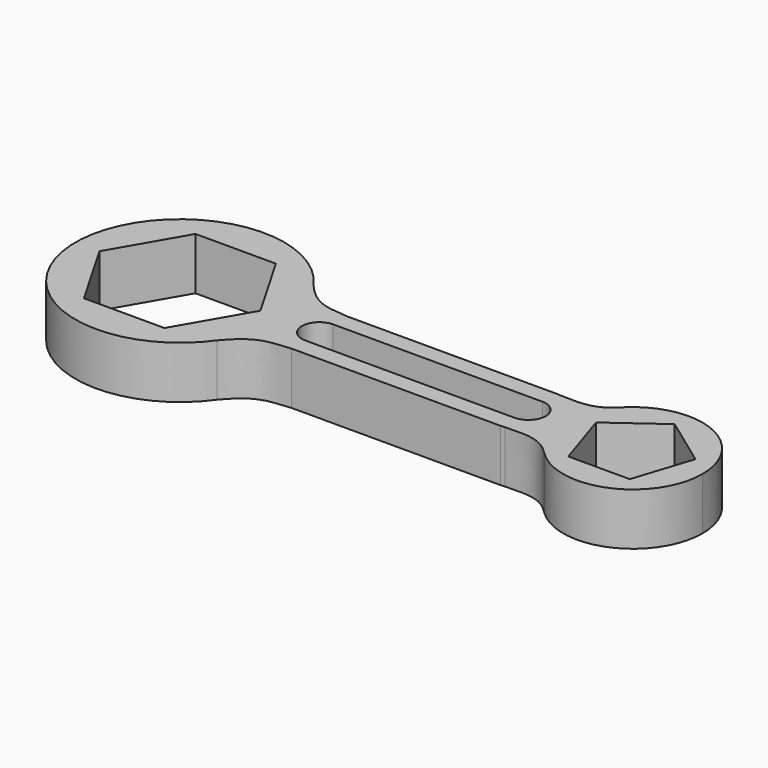
from build123d import *

# Parameters (mm, degrees)
F1_DEPTH = 15


with BuildPart() as f1:
    # F0 (on Top) → F1 (new body)
    with BuildSketch(Plane.XY):
        with BuildLine():
            Line((30, 10), (-30, 10))
            ThreePointArc((-30, 10), (-37.0710678119, 7.0710678119), (-40, 0))
            ThreePointArc((-40, 0), (-37.0710678119, -7.0710678119), (-30, -10))
            Line((-30, -10), (30, -10))
            add(Edge.make_bspline(
                [(30, -10), (30.4419813549, -9.9690694458), (30.8687106597, -9.941549094), (31.2810670558, -9.9176039041)],
                knots=[0, 0, 0, 0, 0.775534817, 0.775534817, 0.775534817, 0.775534817], degree=3))
            ThreePointArc((31.2810670558, -9.9176039041), (37.51034856, -6.6026255768), (40, 4.32e-08))
            ThreePointArc((40, 4.32e-08), (37.5103485315, 6.6026256092), (31.2810670558, 9.9176039041))
            add(Edge.make_bspline(
                [(30, 10), (30.4419813549, 9.9690694458), (30.8687106597, 9.941549094), (31.2810670558, 9.9176039041)],
                knots=[0, 0, 0, 0, 0.775534817, 0.775534817, 0.775534817, 0.775534817], degree=3))
        make_face()
        with BuildLine():
            Line((30, -5), (-30, -5))
            ThreePointArc((-30, -5), (-35, 0), (-30, 5))
            Line((-30, 5), (30, 5))
            ThreePointArc((30, 5), (35, 0), (30, -5))
        make_face(mode=Mode.SUBTRACT)
        with BuildLine():
            ThreePointArc((-40, 0), (-37.0710678119, 7.0710678119), (-30, 10))
            add(Edge.make_bspline(
                [(-30, 10), (-36.5690253675, 10.6094982475), (-39.7284552455, 10.459353216), (-45.5274550985, 17.3520761307)],
                knots=[0, 0, 0, 0, 17.1800723301, 17.1800723301, 17.1800723301, 17.1800723301], degree=3))
            ThreePointArc((-45.5274550985, 17.3520761307), (-41.4152457852, 9.1055931426), (-40, 0))
        make_face()
        with BuildLine():
            ThreePointArc((-45.5274550985, -17.3520761307), (-41.4152457852, -9.1055931426), (-40, 0))
            ThreePointArc((-40, 0), (-41.4152457852, 9.1055931426), (-45.5274550985, 17.3520761307))
            ThreePointArc((-45.5274550985, 17.3520761307), (-100, 0), (-45.5274550985, -17.3520761307))
        make_face()
        Polygon((-93.0940107676, 0), (-81.5470053838, 20), (-58.4529946162, 20), (-46.9059892324, 0), (-58.4529946162, -20), (-81.5470053838, -20), align=None, mode=Mode.SUBTRACT)
        with BuildLine():
            ThreePointArc((-30, -10), (-37.0710678119, -7.0710678119), (-40, 0))
            ThreePointArc((-40, 0), (-41.4152457852, -9.1055931426), (-45.5274550985, -17.3520761307))
            add(Edge.make_bspline(
                [(-30, -10), (-36.5690253675, -10.6094982475), (-39.7284552455, -10.459353216), (-45.5274550985, -17.3520761307)],
                knots=[0, 0, 0, 0, 17.1800723301, 17.1800723301, 17.1800723301, 17.1800723301], degree=3))
        make_face()
        with BuildLine():
            add(Edge.make_bspline(
                [(31.2810670558, 9.9176039041), (39.496869131, 9.4405191711), (42.0070999801, 10.3826559201), (45.765051322, 14.0487094117)],
                knots=[0.775534817, 0.775534817, 0.775534817, 0.775534817, 16.2273154098, 16.2273154098, 16.2273154098, 16.2273154098], degree=3))
            ThreePointArc((31.2810670558, 9.9176039041), (37.5103485315, 6.6026256092), (40, 4.32e-08))
            ThreePointArc((40, 4.32e-08), (41.4973113717, 7.5927935257), (45.765051322, 14.0487094117))
        make_face()
        with BuildLine():
            ThreePointArc((45.765051322, -14.0487094117), (41.4973113553, -7.5927934857), (40, 4.32e-08))
            ThreePointArc((40, 4.32e-08), (37.51034856, -6.6026255768), (31.2810670558, -9.9176039041))
            add(Edge.make_bspline(
                [(31.2810670558, -9.9176039041), (39.496869131, -9.4405191711), (42.0070999801, -10.3826559201), (45.765051322, -14.0487094117)],
                knots=[0.775534817, 0.775534817, 0.775534817, 0.775534817, 16.2273154098, 16.2273154098, 16.2273154098, 16.2273154098], degree=3))
        make_face()
        with BuildLine():
            ThreePointArc((45.765051322, 14.0487094117), (41.4973113717, 7.5927935257), (40, 4.32e-08))
            ThreePointArc((40, 4.32e-08), (41.4973113553, -7.5927934857), (45.765051322, -14.0487094117))
            add(Edge.make_bspline(
                [(45.765051322, -14.0487094117), (45.8848721077, -14.1656000709), (46.0059613608, -14.2852599399), (46.1285444707, -14.4077313099)],
                knots=[16.2273154098, 16.2273154098, 16.2273154098, 16.2273154098, 16.7199892956, 16.7199892956, 16.7199892956, 16.7199892956], degree=3))
            ThreePointArc((46.1285444707, -14.4077313099), (67.828502073, -18.4041993929), (80, 0))
            ThreePointArc((80, 0), (67.828502073, 18.4041993929), (46.1285444707, 14.4077313099))
            add(Edge.make_bspline(
                [(45.765051322, 14.0487094117), (45.8848721077, 14.1656000709), (46.0059613608, 14.2852599399), (46.1285444707, 14.4077313099)],
                knots=[16.2273154098, 16.2273154098, 16.2273154098, 16.2273154098, 16.7199892956, 16.7199892956, 16.7199892956, 16.7199892956], degree=3))
        make_face()
        Polygon((45.7341522556, 4.6352549156), (60, 15), (74.2658477444, 4.6352549156), (68.8167787844, -12.1352549156), (51.1832212156, -12.1352549156), align=None, mode=Mode.SUBTRACT)
    extrude(amount=F1_DEPTH)


solid = f1.part
